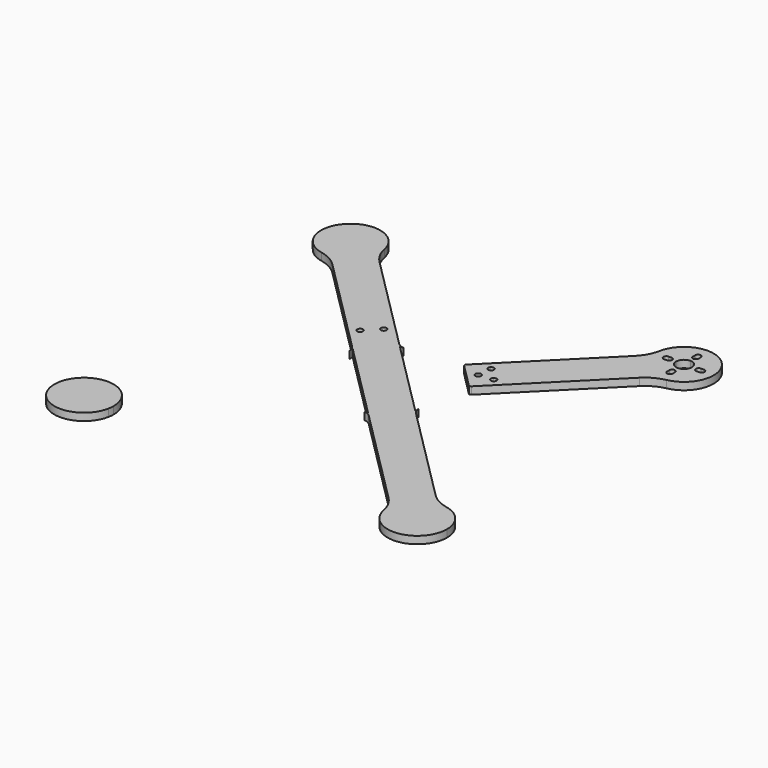
from build123d import *

# Parameters (mm, degrees)
F1_DEPTH = 4


# Not quite as in the source:
# - a feature names something its author has since deleted; it is built from what else it names


with BuildPart() as f1:
    # F0 (on Top) → F1 (new body)
    with BuildSketch(Plane.XY):
        with BuildLine():
            Line((36.2053791718, 68.1711297919), (41.1553791718, 68.1711297919))
            ThreePointArc((41.1553791718, 68.1711297919), (36.4690876708, 79.4848382909), (25.1553791718, 84.1711297919))
            Line((25.1553791718, 84.1711297919), (25.1553791718, 79.2211297919))
            ThreePointArc((25.1553791718, 79.2211297919), (26.2513946827, 78.7671453027), (26.7053791718, 77.6711297919))
            Line((26.7053791718, 77.6711297919), (26.7053791718, 76.1711297919))
            ThreePointArc((26.7053791718, 76.1711297919), (26.2513946827, 75.075114281), (25.1553791718, 74.6211297919))
            Line((25.1553791718, 74.6211297919), (25.1553791718, 72.4211297919))
            ThreePointArc((25.1553791718, 72.4211297919), (28.1605829919, 71.1763336119), (29.4053791718, 68.1711297919))
            Line((29.4053791718, 68.1711297919), (31.6053791718, 68.1711297919))
            ThreePointArc((31.6053791718, 68.1711297919), (32.059363661, 69.2671453027), (33.1553791718, 69.7211297919))
            Line((33.1553791718, 69.7211297919), (34.6553791718, 69.7211297919))
            ThreePointArc((34.6553791718, 69.7211297919), (35.7513946827, 69.2671453027), (36.2053791718, 68.1711297919))
        make_face()
        with BuildLine():
            ThreePointArc((28.3295819531, 52.4891517054), (37.5405970645, 58.041649166), (41.1553791718, 68.1711297919))
            Line((41.1553791718, 68.1711297919), (36.2053791718, 68.1711297919))
            ThreePointArc((36.2053791718, 68.1711297919), (35.7513946827, 67.075114281), (34.6553791718, 66.6211297919))
            Line((34.6553791718, 66.6211297919), (33.1553791718, 66.6211297919))
            ThreePointArc((33.1553791718, 66.6211297919), (32.059363661, 67.075114281), (31.6053791718, 68.1711297919))
            Line((31.6053791718, 68.1711297919), (29.4053791718, 68.1711297919))
            ThreePointArc((29.4053791718, 68.1711297919), (28.1605829919, 65.1659259718), (25.1553791718, 63.9211297919))
            Line((25.1553791718, 63.9211297919), (25.1553791718, 61.7211297919))
            ThreePointArc((25.1553791718, 61.7211297919), (26.2513946827, 61.2671453027), (26.7053791718, 60.1711297919))
            Line((26.7053791718, 60.1711297919), (26.7053791718, 58.6711297919))
            ThreePointArc((26.7053791718, 58.6711297919), (26.2513946827, 57.575114281), (25.1553791718, 57.1211297919))
            Line((25.1553791718, 57.1211297919), (25.1553791718, 52.1711297919))
            ThreePointArc((25.1553791718, 52.1711297919), (26.7504262898, 52.250833793), (28.3295819531, 52.4891517054))
        make_face()
        with BuildLine():
            Line((25.1553791718, 79.2211297919), (25.1553791718, 84.1711297919))
            ThreePointArc((25.1553791718, 84.1711297919), (15.0258985265, 80.5563476687), (9.4734010754, 71.3453325238))
            ThreePointArc((9.4734010754, 71.3453325238), (9.2350831705, 69.7661768848), (9.1553791718, 68.1711297919))
            Line((9.1553791718, 68.1711297919), (14.1053791718, 68.1711297919))
            ThreePointArc((14.1053791718, 68.1711297919), (14.559363661, 69.2671453027), (15.6553791718, 69.7211297919))
            Line((15.6553791718, 69.7211297919), (17.1553791718, 69.7211297919))
            ThreePointArc((17.1553791718, 69.7211297919), (18.2513946827, 69.2671453027), (18.7053791718, 68.1711297919))
            Line((18.7053791718, 68.1711297919), (20.9053791718, 68.1711297919))
            ThreePointArc((20.9053791718, 68.1711297919), (22.1501753518, 71.1763336119), (25.1553791718, 72.4211297919))
            Line((25.1553791718, 72.4211297919), (25.1553791718, 74.6211297919))
            ThreePointArc((25.1553791718, 74.6211297919), (24.059363661, 75.075114281), (23.6053791718, 76.1711297919))
            Line((23.6053791718, 76.1711297919), (23.6053791718, 77.6711297919))
            ThreePointArc((23.6053791718, 77.6711297919), (24.059363661, 78.7671453027), (25.1553791718, 79.2211297919))
        make_face()
        with BuildLine():
            ThreePointArc((18.1552000116, 47.0288150079), (22.8397544367, 50.5092261028), (28.3295819531, 52.4891517054))
            ThreePointArc((28.3295819531, 52.4891517054), (26.7504262898, 52.250833793), (25.1553791718, 52.1711297919))
            ThreePointArc((25.1553791718, 52.1711297919), (24.273692961, 52.1954410923), (23.3946861174, 52.2683011137))
            Line((23.3946861174, 52.2683011137), (18.1552000116, 47.0288150079))
        make_face()
        with BuildLine():
            ThreePointArc((9.1553791718, 68.1711297919), (9.2350831705, 69.7661768848), (9.4734010754, 71.3453325238))
            ThreePointArc((9.4734010754, 71.3453325238), (7.4934752577, 65.8555046373), (4.0130637502, 61.170949994))
            Line((4.0130637502, 61.170949994), (9.2525504936, 66.4104367374))
            ThreePointArc((9.2525504936, 66.4104367374), (9.1796904723, 67.289443581), (9.1553791718, 68.1711297919))
        make_face()
        with BuildLine():
            ThreePointArc((23.3946861174, 52.2683011137), (24.273692961, 52.1954410923), (25.1553791718, 52.1711297919))
            Line((25.1553791718, 52.1711297919), (25.1553791718, 57.1211297919))
            ThreePointArc((25.1553791718, 57.1211297919), (24.059363661, 57.575114281), (23.6053791718, 58.6711297919))
            Line((23.6053791718, 58.6711297919), (23.6053791718, 60.1711297919))
            ThreePointArc((23.6053791718, 60.1711297919), (24.059363661, 61.2671453027), (25.1553791718, 61.7211297919))
            Line((25.1553791718, 61.7211297919), (25.1553791718, 63.9211297919))
            ThreePointArc((25.1553791718, 63.9211297919), (23.5289745843, 64.2446417787), (22.1501753518, 65.1659259718))
            Line((22.1501753518, 65.1659259718), (13.8416706728, 56.8574212929))
            ThreePointArc((13.8416706728, 56.8574212929), (18.2271759416, 53.74892469), (23.3946861174, 52.2683011137))
        make_face()
        with BuildLine():
            Line((-20.2968936134, 8.5767213829), (18.1552000116, 47.0288150079))
            Line((18.1552000116, 47.0288150079), (23.3946861174, 52.2683011137))
            ThreePointArc((23.3946861174, 52.2683011137), (18.2271759416, 53.74892469), (13.8416706728, 56.8574212929))
            Line((13.8416706728, 56.8574212929), (-27.3679614253, 15.6477891948))
            Line((-27.3679614253, 15.6477891948), (-20.2968936134, 8.5767213829))
        make_face()
        with BuildLine():
            Line((14.1053791718, 68.1711297919), (9.1553791718, 68.1711297919))
            ThreePointArc((9.1553791718, 68.1711297919), (9.1796904723, 67.289443581), (9.2525504936, 66.4104367374))
            ThreePointArc((9.2525504936, 66.4104367374), (10.73317407, 61.2429265616), (13.8416706728, 56.8574212929))
            Line((13.8416706728, 56.8574212929), (22.1501753518, 65.1659259718))
            ThreePointArc((22.1501753518, 65.1659259718), (21.2288911587, 66.5447252043), (20.9053791718, 68.1711297919))
            Line((20.9053791718, 68.1711297919), (18.7053791718, 68.1711297919))
            ThreePointArc((18.7053791718, 68.1711297919), (18.2513946827, 67.075114281), (17.1553791718, 66.6211297919))
            Line((17.1553791718, 66.6211297919), (15.6553791718, 66.6211297919))
            ThreePointArc((15.6553791718, 66.6211297919), (14.559363661, 67.075114281), (14.1053791718, 68.1711297919))
        make_face()
        with BuildLine():
            Line((9.2525504936, 66.4104367374), (4.0130637502, 61.170949994))
            Line((4.0130637502, 61.170949994), (-34.4390292371, 22.7188570066))
            Line((-34.4390292371, 22.7188570066), (-27.3679614253, 15.6477891948))
            Line((-27.3679614253, 15.6477891948), (13.8416706728, 56.8574212929))
            ThreePointArc((13.8416706728, 56.8574212929), (10.73317407, 61.2429265616), (9.2525504936, 66.4104367374))
        make_face()
        with BuildLine():
            Line((-25.2466410817, 3.6269739146), (-20.2968936134, 8.5767213829))
            Line((-20.2968936134, 8.5767213829), (-27.3679614253, 15.6477891948))
            Line((-27.3679614253, 15.6477891948), (-32.3177088936, 10.6980417265))
            Line((-32.3177088936, 10.6980417265), (-29.8781904985, 8.2585233314))
            ThreePointArc((-29.8781904985, 8.2585233314), (-28.1890156675, 8.5945210959), (-27.2321749877, 7.1625078205))
            ThreePointArc((-27.2321749877, 7.1625078205), (-27.3501617123, 6.5693485004), (-27.6861594768, 6.0664923097))
            Line((-27.6861594768, 6.0664923097), (-25.2466410817, 3.6269739146))
        make_face()
        with BuildLine():
            Line((-27.3679614253, 15.6477891948), (-34.4390292371, 22.7188570066))
            Line((-34.4390292371, 22.7188570066), (-39.3887767054, 17.7691095383))
            Line((-39.3887767054, 17.7691095383), (-36.9492583104, 15.3295911432))
            ThreePointArc((-36.9492583104, 15.3295911432), (-35.2600834794, 15.6655889078), (-34.3032427995, 14.2335756324))
            ThreePointArc((-34.3032427995, 14.2335756324), (-34.4212295241, 13.6404163122), (-34.7572272887, 13.1375601216))
            Line((-34.7572272887, 13.1375601216), (-32.3177088936, 10.6980417265))
            Line((-32.3177088936, 10.6980417265), (-27.3679614253, 15.6477891948))
        make_face()
        with BuildLine():
            Line((-32.3177088936, -3.4440938973), (-25.2466410817, 3.6269739146))
            Line((-25.2466410817, 3.6269739146), (-27.6861594768, 6.0664923097))
            ThreePointArc((-27.6861594768, 6.0664923097), (-29.8781904985, 6.0664923097), (-29.8781904985, 8.2585233314))
            Line((-29.8781904985, 8.2585233314), (-32.3177088936, 10.6980417265))
            Line((-32.3177088936, 10.6980417265), (-35.4643340699, 7.5514165502))
            ThreePointArc((-35.4643340699, 7.5514165502), (-35.1283363053, 7.0485603595), (-35.0103495807, 6.4554010393))
            ThreePointArc((-35.0103495807, 6.4554010393), (-35.9671902605, 5.023387764), (-37.6563650915, 5.3593855285))
            Line((-37.6563650915, 5.3593855285), (-40.0958834866, 2.9198671334))
            Line((-40.0958834866, 2.9198671334), (-33.731922456, -3.4440938973))
            ThreePointArc((-33.731922456, -3.4440938973), (-33.0248156748, -3.7369871161), (-32.3177088936, -3.4440938973))
        make_face()
        with BuildLine():
            Line((-36.9492583104, 15.3295911432), (-39.3887767054, 17.7691095383))
            Line((-39.3887767054, 17.7691095383), (-46.4598445173, 10.6980417265))
            ThreePointArc((-46.4598445173, 10.6980417265), (-46.7527377361, 9.9909349453), (-46.4598445173, 9.2838281641))
            Line((-46.4598445173, 9.2838281641), (-40.0958834866, 2.9198671334))
            Line((-40.0958834866, 2.9198671334), (-37.6563650915, 5.3593855285))
            ThreePointArc((-37.6563650915, 5.3593855285), (-37.6563650915, 7.5514165502), (-35.4643340699, 7.5514165502))
            Line((-35.4643340699, 7.5514165502), (-32.3177088936, 10.6980417265))
            Line((-32.3177088936, 10.6980417265), (-34.7572272887, 13.1375601216))
            ThreePointArc((-34.7572272887, 13.1375601216), (-36.9492583104, 13.1375601216), (-36.9492583104, 15.3295911432))
        make_face()
    extrude(amount=F1_DEPTH)


with BuildPart() as f1b:
    # F0 (on Top) → F1, piece 2 (new body)
    with BuildSketch(Plane.XY):
        with BuildLine():
            ThreePointArc((-138.8446208282, -111.8288702081), (-140.062548308, -105.7059352903), (-143.5309123292, -100.5151617091))
            ThreePointArc((-143.5309123292, -100.5151617091), (-150.2258187408, -96.5100364641), (-158.0188236998, -96.14689214))
            ThreePointArc((-158.0188236998, -96.14689214), (-166.1583293272, -123.1425787071), (-139.16264276, -115.0030730797))
            ThreePointArc((-139.16264276, -115.0030730797), (-138.9243248339, -113.4239173719), (-138.8446208282, -111.8288702081))
        make_face()
    extrude(amount=F1_DEPTH)


with BuildPart() as f1c:
    # F0 (on Top) → F1, piece 3 (new body)
    with BuildSketch(Plane.XY):
        Polygon((-50.7024852044, -21.8288702081), (-57.7735530163, -14.7578023963), (-64.8446208282, -21.8288702081), align=None)
        Polygon((-64.8446208282, -21.8288702081), (-57.7735530163, -14.7578023963), (-64.8446208282, -7.6867345844), align=None)
        Polygon((-78.9867564519, -21.8288702081), (-64.8446208282, -21.8288702081), (-89.5933581697, 2.9198671334), (-96.6644259816, -4.1512006785), (-94.3090869492, -6.5065397108), (-92.8446208282, -7.9710058318), align=None)
        with BuildLine():
            Line((-50.7024852044, -21.8288702081), (-64.8446208282, -21.8288702081))
            Line((-64.8446208282, -21.8288702081), (13.8416706728, -100.5151617091))
            ThreePointArc((13.8416706728, -100.5151617091), (18.2271759416, -97.4066651063), (23.3946861174, -95.9260415299))
            Line((23.3946861174, -95.9260415299), (18.1551993662, -90.6865547787))
            Line((18.1551993662, -90.6865547787), (-35.3801547186, -37.151200694))
            Line((-35.3801547186, -37.151200694), (-36.8446208282, -35.6867345844))
            Line((-36.8446208282, -35.6867345844), (-50.7024852044, -21.8288702081))
        make_face()
        Polygon((-64.8446208282, -35.9710058318), (-64.8446208282, -21.8288702081), (-71.91568864, -28.89993802), align=None)
        Polygon((-89.5933581697, 2.9198671334), (-64.8446208282, -21.8288702081), (-64.8446208282, -7.6867345844), (-78.7024852044, 6.1711297919), (-80.1669513924, 7.6355959798), (-82.5222903578, 9.9909349453), align=None)
        with BuildLine():
            Line((13.8416706728, -100.5151617091), (-64.8446208282, -21.8288702081))
            Line((-64.8446208282, -21.8288702081), (-64.8446208282, -35.9710058318))
            Line((-64.8446208282, -35.9710058318), (-50.9867564519, -49.8288702081))
            Line((-50.9867564519, -49.8288702081), (-49.5222903639, -51.2933362961))
            Line((-49.5222903639, -51.2933362961), (4.0130642277, -104.8286908877))
            Line((4.0130642277, -104.8286908877), (9.2525504936, -110.0681771537))
            ThreePointArc((9.2525504936, -110.0681771537), (10.73317407, -104.9006669778), (13.8416706728, -100.5151617091))
        make_face()
        Polygon((-71.91568864, -28.89993802), (-64.8446208282, -21.8288702081), (-78.9867564519, -21.8288702081), align=None)
        with BuildLine():
            Line((-96.6644259816, -4.1512006785), (-89.5933581697, 2.9198671334))
            Line((-89.5933581697, 2.9198671334), (-92.0328765648, 5.3593855285))
            ThreePointArc((-92.0328765648, 5.3593855285), (-94.2249075865, 5.3593855285), (-94.2249075865, 7.5514165502))
            Line((-94.2249075865, 7.5514165502), (-97.3715327627, 10.6980417265))
            Line((-97.3715327627, 10.6980417265), (-99.8110511578, 8.2585233314))
            ThreePointArc((-99.8110511578, 8.2585233314), (-99.4750533933, 7.7556671407), (-99.3570666687, 7.1625078205))
            ThreePointArc((-99.3570666687, 7.1625078205), (-100.3139073485, 5.7304945451), (-102.0030821795, 6.0664923097))
            Line((-102.0030821795, 6.0664923097), (-104.4426005746, 3.6269739146))
            Line((-104.4426005746, 3.6269739146), (-96.6644259816, -4.1512006785))
        make_face()
        with BuildLine():
            Line((-92.0328765648, 5.3593855285), (-89.5933581697, 2.9198671334))
            Line((-89.5933581697, 2.9198671334), (-82.5222903578, 9.9909349453))
            Line((-82.5222903578, 9.9909349453), (-90.3004649509, 17.7691095383))
            Line((-90.3004649509, 17.7691095383), (-92.739983346, 15.3295911432))
            ThreePointArc((-92.739983346, 15.3295911432), (-92.4039855814, 14.8267349526), (-92.2859988568, 14.2335756324))
            ThreePointArc((-92.2859988568, 14.2335756324), (-93.2428395366, 12.801562357), (-94.9320143677, 13.1375601216))
            Line((-94.9320143677, 13.1375601216), (-97.3715327627, 10.6980417265))
            Line((-97.3715327627, 10.6980417265), (-94.2249075865, 7.5514165502))
            ThreePointArc((-94.2249075865, 7.5514165502), (-92.5357327555, 7.8874143147), (-91.5788920756, 6.4554010393))
            ThreePointArc((-91.5788920756, 6.4554010393), (-91.6968788002, 5.8622417192), (-92.0328765648, 5.3593855285))
        make_face()
        with BuildLine():
            ThreePointArc((23.3946861174, -95.9260415299), (18.2271759416, -97.4066651063), (13.8416706728, -100.5151617091))
            ThreePointArc((13.8416706728, -100.5151617091), (10.73317407, -104.9006669778), (9.2525504936, -110.0681771537))
            ThreePointArc((9.2525504936, -110.0681771537), (9.1713776761, -112.5441996308), (9.4734010854, -115.0030729893))
            ThreePointArc((9.4734010854, -115.0030729893), (26.7504262898, -127.749166207), (41.1553791718, -111.8288702081))
            ThreePointArc((41.1553791718, -111.8288702081), (37.5405969765, -101.6993894746), (28.3295816805, -96.1468920665))
            ThreePointArc((28.3295816805, -96.1468920665), (25.8707084556, -95.8448687061), (23.3946861174, -95.9260415299))
        make_face()
        with BuildLine():
            Line((-80.1669513924, 7.6355959798), (-78.7024852044, 6.1711297919))
            Line((-78.7024852044, 6.1711297919), (-76.6314173926, 6.1711297919))
            ThreePointArc((-76.6314173926, 6.1711297919), (-78.5448346157, 6.5517321547), (-80.1669513924, 7.6355959798))
        make_face()
        with BuildLine():
            Line((-36.8446208282, -33.6156667725), (-36.8446208282, -35.6867345844))
            Line((-36.8446208282, -35.6867345844), (-35.3801547186, -37.151200694))
            ThreePointArc((-35.3801547186, -37.151200694), (-36.4640184865, -35.5290839445), (-36.8446208282, -33.6156667725))
        make_face()
        with BuildLine():
            ThreePointArc((-94.2249075865, 7.5514165502), (-94.2249075865, 5.3593855285), (-92.0328765648, 5.3593855285))
            Line((-92.0328765648, 5.3593855285), (-94.2249075865, 7.5514165502))
        make_face()
        with BuildLine():
            Line((-94.2249075865, 7.5514165502), (-92.0328765648, 5.3593855285))
            ThreePointArc((-92.0328765648, 5.3593855285), (-91.6968788002, 5.8622417192), (-91.5788920756, 6.4554010393))
            ThreePointArc((-91.5788920756, 6.4554010393), (-92.5357327555, 7.8874143147), (-94.2249075865, 7.5514165502))
        make_face()
        with BuildLine():
            Line((18.1551993662, -90.6865547787), (23.3946861174, -95.9260415299))
            ThreePointArc((23.3946861174, -95.9260415299), (25.8707084556, -95.8448687061), (28.3295816805, -96.1468920665))
            ThreePointArc((28.3295816805, -96.1468920665), (22.839753912, -94.1669662375), (18.1551993662, -90.6865547787))
        make_face()
        with BuildLine():
            ThreePointArc((9.4734010854, -115.0030729893), (9.1713776761, -112.5441996308), (9.2525504936, -110.0681771537))
            Line((9.2525504936, -110.0681771537), (4.0130642277, -104.8286908877))
            ThreePointArc((4.0130642277, -104.8286908877), (7.4934754292, -109.5132453732), (9.4734010854, -115.0030729893))
        make_face()
        with BuildLine():
            Line((-49.5222903639, -51.2933362961), (-50.9867564519, -49.8288702081))
            Line((-50.9867564519, -49.8288702081), (-53.0578242638, -49.8288702081))
            ThreePointArc((-53.0578242638, -49.8288702081), (-51.1444071059, -50.2094725439), (-49.5222903639, -51.2933362961))
        make_face()
        with BuildLine():
            Line((-92.8446208282, -10.0420736437), (-92.8446208282, -7.9710058318))
            Line((-92.8446208282, -7.9710058318), (-94.3090869492, -6.5065397108))
            ThreePointArc((-94.3090869492, -6.5065397108), (-93.2252231729, -8.1286564643), (-92.8446208282, -10.0420736437))
        make_face()
        with BuildLine():
            Line((-109.3923480429, 8.5767213829), (-104.4426005746, 3.6269739146))
            Line((-104.4426005746, 3.6269739146), (-102.0030821795, 6.0664923097))
            ThreePointArc((-102.0030821795, 6.0664923097), (-102.0030821795, 8.2585233314), (-99.8110511578, 8.2585233314))
            Line((-99.8110511578, 8.2585233314), (-97.3715327627, 10.6980417265))
            Line((-97.3715327627, 10.6980417265), (-102.3212802311, 15.6477891948))
            Line((-102.3212802311, 15.6477891948), (-109.3923480429, 8.5767213829))
        make_face()
        with BuildLine():
            Line((-92.739983346, 15.3295911432), (-90.3004649509, 17.7691095383))
            Line((-90.3004649509, 17.7691095383), (-95.2502124192, 22.7188570066))
            Line((-95.2502124192, 22.7188570066), (-102.3212802311, 15.6477891948))
            Line((-102.3212802311, 15.6477891948), (-97.3715327627, 10.6980417265))
            Line((-97.3715327627, 10.6980417265), (-94.9320143677, 13.1375601216))
            ThreePointArc((-94.9320143677, 13.1375601216), (-94.9320143677, 15.3295911432), (-92.739983346, 15.3295911432))
        make_face()
        with BuildLine():
            Line((-147.8444409361, 47.0288142761), (-109.3923480429, 8.5767213829))
            Line((-109.3923480429, 8.5767213829), (-102.3212802311, 15.6477891948))
            Line((-102.3212802311, 15.6477891948), (-143.5309123292, 56.8574212929))
            ThreePointArc((-143.5309123292, 56.8574212929), (-147.9164175979, 53.74892469), (-153.0839277737, 52.2683011137))
            Line((-153.0839277737, 52.2683011137), (-147.8444409361, 47.0288142761))
        make_face()
        with BuildLine():
            Line((-102.3212802311, 15.6477891948), (-95.2502124192, 22.7188570066))
            Line((-95.2502124192, 22.7188570066), (-133.7023062703, 61.1709508578))
            Line((-133.7023062703, 61.1709508578), (-138.94179215, 66.4104367374))
            ThreePointArc((-138.94179215, 66.4104367374), (-140.4224157263, 61.2429265616), (-143.5309123292, 56.8574212929))
            Line((-143.5309123292, 56.8574212929), (-102.3212802311, 15.6477891948))
        make_face()
        with BuildLine():
            ThreePointArc((-158.0188232221, 52.4891516271), (-152.528995463, 50.5092257647), (-147.8444409361, 47.0288142761))
            Line((-147.8444409361, 47.0288142761), (-153.0839277737, 52.2683011137))
            ThreePointArc((-153.0839277737, 52.2683011137), (-155.5599500534, 52.1871282873), (-158.0188232221, 52.4891516271))
        make_face()
        with BuildLine():
            Line((-138.94179215, 66.4104367374), (-133.7023062703, 61.1709508578))
            ThreePointArc((-133.7023062703, 61.1709508578), (-137.1827173467, 65.8555054434), (-139.1626428524, 71.3453331199))
            ThreePointArc((-139.1626428524, 71.3453331199), (-138.9243248571, 69.7661771874), (-138.8446208282, 68.1711297919))
            ThreePointArc((-138.8446208282, 68.1711297919), (-138.8689321286, 67.289443581), (-138.94179215, 66.4104367374))
        make_face()
        with BuildLine():
            ThreePointArc((-153.0839277737, 52.2683011137), (-147.9164175979, 53.74892469), (-143.5309123292, 56.8574212929))
            ThreePointArc((-143.5309123292, 56.8574212929), (-140.4224157263, 61.2429265616), (-138.94179215, 66.4104367374))
            ThreePointArc((-138.94179215, 66.4104367374), (-138.8689321286, 67.289443581), (-138.8446208282, 68.1711297919))
            ThreePointArc((-138.8446208282, 68.1711297919), (-138.9243248571, 69.7661771874), (-139.1626428524, 71.3453331199))
            ThreePointArc((-139.1626428524, 71.3453331199), (-166.1583296641, 79.4848379539), (-158.0188232221, 52.4891516271))
            ThreePointArc((-158.0188232221, 52.4891516271), (-155.5599500534, 52.1871282873), (-153.0839277737, 52.2683011137))
        make_face()
    extrude(amount=F1_DEPTH)


solid = Compound([f1.part, f1b.part, f1c.part])
